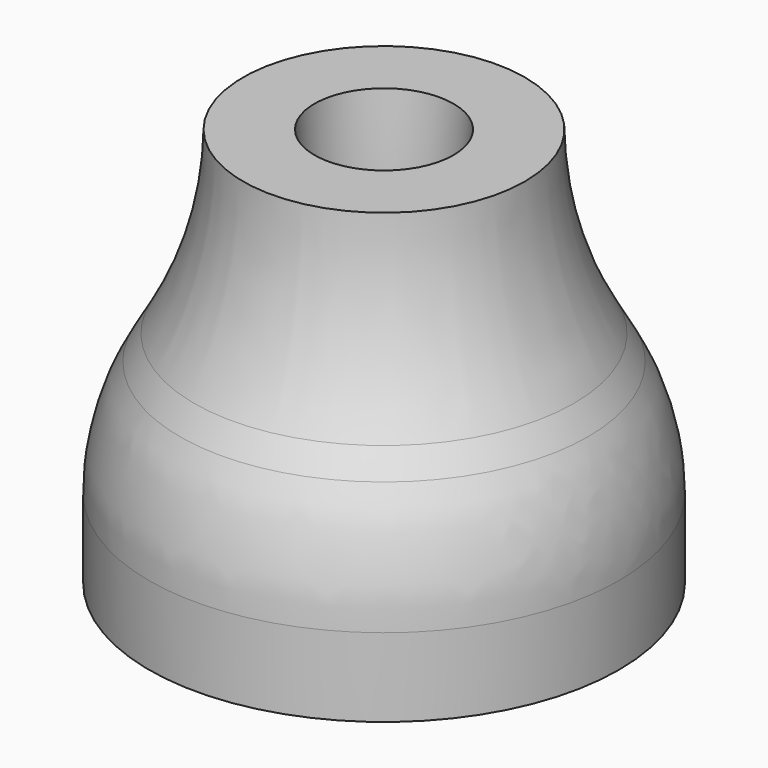
from build123d import *

# Parameters (mm, degrees)
F2_R     = 5
F3_DEPTH = 2
F4_SIZE  = 0.1


# Not quite as in the source:
# - a fillet or chamfer that OpenCascade refuses, or shapes differently, is made with other operations: its cross-section is extruded or revolved along the edge and cut away or added


with BuildPart() as f1:
    # F0 (on Front) → F1 (revolve)
    with BuildSketch(Plane.XZ):
        Polygon((0, 3), (0, 0), (5, 0), (5, 3), (3, 6.4998515683), (1.38, 6.4998515683), (1.38, 3), align=None)
    revolve(axis=Axis((0, 0, 4.7499257841), (0, 0, 1)))

    # F2
    f2_edges = [f1.edges().sort_by_distance(p)[0] for p in [
        (-5, 0, 3),
    ]]
    fillet(f2_edges, radius=F2_R)

    # F3 (add): a face of the model
    f3_faces = [f1.faces().sort_by_distance(p)[0] for p in [
        (-2.9151471863, 0, 6.4998515683),
    ]]
    extrude(f3_faces, amount=F3_DEPTH)

    # F4
    f4_edges = [f1.edges().sort_by_distance(p)[0] for p in [
        (-1.38, 0, 8.499852),
    ]]
    chamfer(f4_edges, length=F4_SIZE)

    # F5: fillet of radius 35 on 1 edges, made by hand

    # F5_s1 → F5_t2 (revolve, cut)
    with BuildSketch(Plane.XZ):
        with BuildLine():
            ThreePointArc((1.48, 8.4998515683), (1.405008935, 7.1788664105), (1.38, 5.8559907549))
            Line((1.38, 5.8559907549), (1.38, 8.3998515683))
            Line((1.38, 8.3998515683), (1.48, 8.4998515683))
        make_face()
    revolve(axis=Axis((0, 0, 8.3998515683), (0, 0, 1)), mode=Mode.SUBTRACT)

    # F6: fillet of radius 7.9 on 1 edges, made by hand

    # F6_s1 → F6_t2 (revolve)
    with BuildSketch(Plane.XZ):
        with BuildLine():
            ThreePointArc((3, 8.4998515683), (3.276921402, 6.5233668652), (4.0403288808, 4.6793532357))
            Line((4.0403288808, 4.6793532357), (3, 6.4998515683))
            Line((3, 6.4998515683), (3, 8.4998515683))
        make_face()
    revolve(axis=Axis((0, 0, 6.4998515683), (0, 0, 1)))


solid = f1.part
